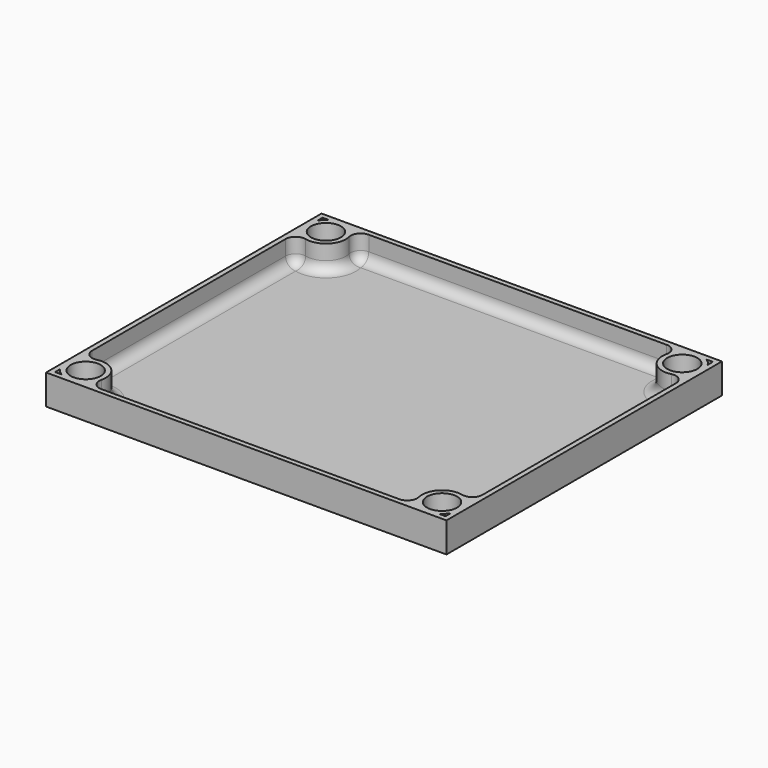
from build123d import *

# Parameters (mm, degrees)
F0_W     = 200
F0_H     = 172
F0_R     = 7.5
F1_DEPTH = 15
F2_T     = 2.5
F3_R     = 5


# Not quite as in the source:
# - a shell that OpenCascade refuses in one call is made with other operations: the cavity is built on its own and cut out


with BuildPart() as f1:
    # F0 (on Top) → F1 (new body)
    with BuildSketch(Plane.XY):
        with Locations((100, 86)):
            Rectangle(F0_W, F0_H)
        with Locations((11, 11)):
            Circle(F0_R, mode=Mode.SUBTRACT)
        with Locations((189, 11)):
            Circle(F0_R, mode=Mode.SUBTRACT)
        with Locations((11, 161)):
            Circle(F0_R, mode=Mode.SUBTRACT)
        with Locations((189, 161)):
            Circle(F0_R, mode=Mode.SUBTRACT)
    extrude(amount=F1_DEPTH)

    # F2: shell of thickness 2.5, made by hand


with BuildPart() as f2_core1:
    # F2_t2: copy of F1
    add(f1.part)

    # the walls: a layer under each face that stays
    f2_faces = [f2_core1.faces().sort_by_distance(p)[0] for p in [
        (0, 86, 7.5),
        (100, 0, 7.5),
        (200, 86, 7.5),
        (100, 172, 7.5),
        (3.5, 11, 7.5),
        (181.5, 11, 7.5),
        (3.5, 161, 7.5),
        (181.5, 161, 7.5),
        (100, 86, 0),
    ]]
    thicken(f2_faces, amount=-F2_T, mode=Mode.SUBTRACT)


with BuildPart() as f1_1:
    add(f1.part)

    # what is left inside the walls is the cavity
    f2_cavity = [f2_core1.part.solids().sort_by_distance(p)[0] for p in [
        (3.911255, 168.088745, 10.833333),
        (100, 58.166667, 14.975),
        (3.911255, 3.911255, 10.833333),
        (196.088745, 168.088745, 10.833333),
        (196.088745, 3.911255, 10.833333),
    ]]
    add(f2_cavity, mode=Mode.SUBTRACT)

    # F3
    f3_edges = [f1_1.edges().sort_by_distance(p)[0] for p in [
        (100, 169.5, 2.5),
        (16.267827, 169.5, 8.75),
        (183.732173, 169.5, 8.75),
        (18.071068, 153.928932, 2.5),
        (2.5, 155.732173, 8.75),
        (2.5, 86, 2.5),
        (2.5, 16.267827, 8.75),
        (18.071068, 18.071068, 2.5),
        (16.267827, 2.5, 8.75),
        (100, 2.5, 2.5),
        (183.732173, 2.5, 8.75),
        (181.928932, 18.071068, 2.5),
        (197.5, 16.267827, 8.75),
        (197.5, 86, 2.5),
        (197.5, 155.732173, 8.75),
        (181.928932, 153.928932, 2.5),
    ]]
    fillet(f3_edges, radius=F3_R)


solid = f1_1.part
